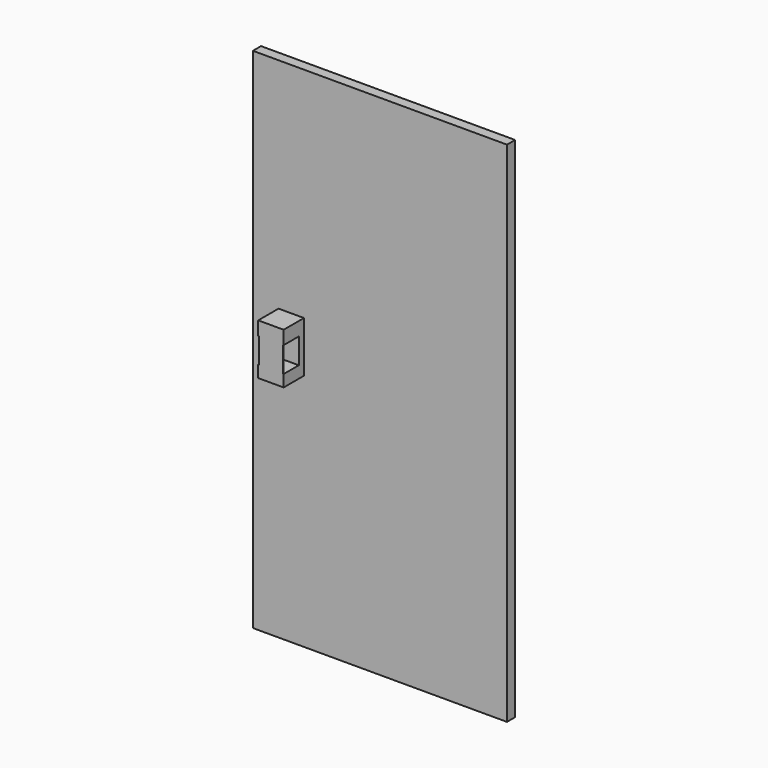
from build123d import *

# Parameters (mm, degrees)
F0_W        = 127
F0_H        = 254
F1_DEPTH    = 2.54
F2_W        = 12.7
F2_H        = 25.4
F3_DEPTH    = 12.7
F4_W        = 6.35
F4_H        = 12.7
F5_DEPTH    = 25.4
F6_T1_DEPTH = 12.7


# Not quite as in the source:
# - a fillet or chamfer that OpenCascade refuses, or shapes differently, is made with other operations: its cross-section is extruded or revolved along the edge and cut away or added


with BuildPart() as f1:
    # F0 (on Front) → F1 (new body, symmetric)
    with BuildSketch(Plane.XZ):
        with Locations((0, -5.0209306781)):
            Rectangle(F0_W, F0_H)
    extrude(amount=F1_DEPTH, both=True)

    # F2 (on face) → F3 (join)
    with BuildSketch(Plane.XZ.offset(2.54)):
        with Locations((-44.3181917071, 0)):
            Rectangle(F2_W, F2_H)
    extrude(amount=F3_DEPTH)

    # F4 (on face) → F5 (cut)
    with BuildSketch(Plane(origin=(-50.6681917071, 0, 0), x_dir=(0, -1, 0), z_dir=(-1, 0, 0))):
        with Locations((8.9468448423, -0.4299022911)):
            Rectangle(F4_W, F4_H)
    extrude(amount=-F5_DEPTH, mode=Mode.SUBTRACT)

    # F6: fillet of radius 5.08 on 2 edges, made by hand

    # F6_s2 → F6_t1 (cut)
    with BuildSketch(Plane.XY.offset(-6.7799022911)):
        with BuildLine():
            ThreePointArc((-50.6681917071, -17.2018448423), (-49.1802941556, -13.6097423939), (-45.5881917071, -12.1218448423))
            Line((-45.5881917071, -12.1218448423), (-50.6681917071, -12.1218448423))
            Line((-50.6681917071, -12.1218448423), (-50.6681917071, -17.2018448423))
        make_face()
        with BuildLine():
            ThreePointArc((-37.9681917071, -17.2018448423), (-39.4560892587, -13.6097423939), (-43.0481917071, -12.1218448423))
            Line((-43.0481917071, -12.1218448423), (-37.9681917071, -12.1218448423))
            Line((-37.9681917071, -12.1218448423), (-37.9681917071, -17.2018448423))
        make_face()
    extrude(amount=F6_T1_DEPTH, mode=Mode.SUBTRACT)


solid = f1.part
